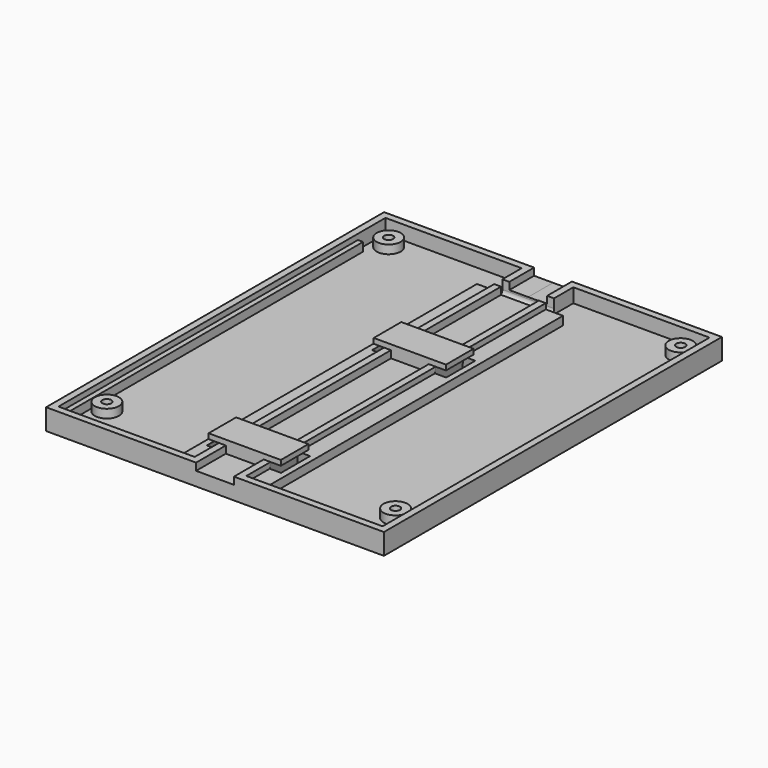
from build123d import *

# Parameters (mm, degrees)
F0_W      = 43.6
F0_H      = 122.8
F1_DEPTH  = 6.1
F2_T      = -2
F3_R      = 3.5
F3_R_2    = 1.3
F4_DEPTH  = 2.5
F5_DEPTH  = 2.001
F6_W      = 1.5
F6_H      = 108.8
F6_W_2    = 5
F7_DEPTH  = 2.5
F8_W      = 5
F8_H      = 10
F9_DEPTH  = 1.5
F10_W     = 3
F10_H     = 10
F11_DEPTH = 25
F11_TAPER = -10
F0_W_2    = 5.5
F12_DEPTH = 4
F14_DEPTH = 15
F16_W     = 10
F16_H     = 3.6
F17_DEPTH = 11


with BuildPart() as f1:
    # F0 (on Top) → F1 (new body)
    with BuildSketch(Plane.XY):
        with Locations((-27.3, 0)):
            Rectangle(F0_W, F0_H)
    extrude(amount=F1_DEPTH)

    # F2
    f2_openings = [f1.faces().sort_by_distance(p)[0] for p in [
        (-27.3, 0, 6.1),
    ]]
    offset(amount=F2_T, openings=f2_openings)

    # F3 (on face) → F4 (join, through all)
    with BuildSketch(Plane.XY.offset(2)):
        with Locations((-42.45, 54.75)):
            Circle(F3_R)
        with Locations((-42.45, 54.75)):
            Circle(F3_R_2, mode=Mode.SUBTRACT)
        with Locations((-41.95, -48.25)):
            Circle(F3_R)
        with Locations((-41.95, -48.25)):
            Circle(F3_R_2, mode=Mode.SUBTRACT)
    extrude(amount=F4_DEPTH)

    # F5 (cut, through all): faces of the model
    f5_faces = [f1.faces().sort_by_distance(p)[0] for p in [
        (-42.45, 54.75, 2),
        (-41.95, -48.25, 2),
    ]]
    extrude(f5_faces, amount=-F5_DEPTH, mode=Mode.SUBTRACT)

    # F6 (on face) → F7 (join, through all)
    with BuildSketch(Plane.XY.offset(2)):
        with Locations((-46.35, -5)):
            Rectangle(F6_W, F6_H)
        with Locations((-10, -5)):
            Rectangle(F6_W_2, F6_H)
    extrude(amount=F7_DEPTH)

    # F8 (on face) → F9 (join)
    with BuildSketch(Plane.XY.offset(6.1)):
        with Locations((-8, 14.4)):
            Rectangle(F8_W, F8_H)
        with Locations((-8, -45.6)):
            Rectangle(F8_W, F8_H)
    extrude(amount=F9_DEPTH)

    # F10 (on face) → F11 (cut)
    with BuildSketch(Plane(origin=(0, 0, 6.1), x_dir=(1, 0, 0), z_dir=(0, 0, -1))):
        with Locations((-9, -14.4)):
            Rectangle(F10_W, F10_H)
        with Locations((-9, 45.6)):
            Rectangle(F10_W, F10_H)
    extrude(amount=F11_DEPTH, taper=F11_TAPER, mode=Mode.SUBTRACT)

    # F0 (on Top) → F12 (join)
    with BuildSketch(Plane.XY):
        with Locations((-2.75, 0)):
            Rectangle(F0_W_2, F0_H)
    extrude(amount=F12_DEPTH)

    # F13 (on face) → F14 (cut)
    with BuildSketch(Plane.YZ):
        with BuildLine():
            Line((49.4, 7), (49.4, 4))
            Line((49.4, 4), (49.4, 3.5))
            ThreePointArc((49.4, 3.5), (50.9, 2), (52.4, 3.5))
            Line((52.4, 3.5), (52.4, 4))
            Line((52.4, 4), (52.4, 7))
            Line((52.4, 7), (49.4, 7))
        make_face()
    extrude(amount=-F14_DEPTH, mode=Mode.SUBTRACT)

    # F15: F1 across plane


with BuildPart() as f1_1:
    add(f1.part)
    add(f1.part.mirror(Plane.YZ))

    # F16 (on face) → F17 (join, through all)
    with BuildSketch(Plane.YZ.offset(-5.5)):
        with Locations((14.4, 5.8)):
            Rectangle(F16_W, F16_H)
        with Locations((-45.6, 5.8)):
            Rectangle(F16_W, F16_H)
    extrude(amount=F17_DEPTH)


solid = f1_1.part
